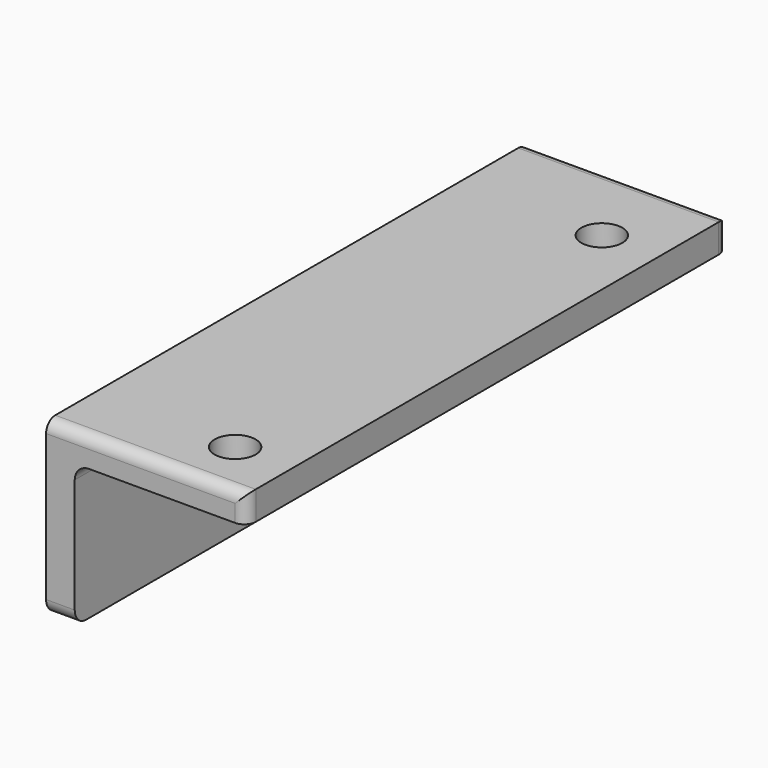
from build123d import *

# Parameters (mm, degrees)
F1_DEPTH = 133.35
F2_R     = 4.5466
F3_DEPTH = 25.4
F4_R     = 4.5466
F5_DEPTH = 25.4
F6_R     = 2.54
F7_R     = 3.175


with BuildPart() as f1:
    # F0 (on Front) → F1 (new body)
    with BuildSketch(Plane.XZ):
        Polygon((-29.6893073604, 12.910717619), (-29.6893073604, -25.189282381), (-23.3393073604, -25.189282381), (-23.3393073604, 6.560717619), (14.7606926396, 6.560717619), (14.7606926396, 12.910717619), align=None)
    extrude(amount=F1_DEPTH)

    # F2 (on face) → F3 (cut)
    with BuildSketch(Plane(origin=(-29.6893073604, 0, 0), x_dir=(0, -1, 0), z_dir=(-1, 0, 0))):
        with Locations((25.4, -14.076782381)):
            Circle(F2_R)
        with Locations((88.9, -14.076782381)):
            Circle(F2_R)
    extrude(amount=-F3_DEPTH, mode=Mode.SUBTRACT)

    # F4 (on face) → F5 (cut)
    with BuildSketch(Plane.XY.offset(12.910717619)):
        with Locations((2.0606926396, -120.65)):
            Circle(F4_R)
        with Locations((2.0606926396, -19.05)):
            Circle(F4_R)
    extrude(amount=-F5_DEPTH, mode=Mode.SUBTRACT)

    # F6
    f6_edges = [f1.edges().sort_by_distance(p)[0] for p in [
        (14.760693, -133.35, 9.735718),
        (-7.464307, -133.35, 12.910718),
        (-7.464307, 0, 12.910718),
        (14.760693, 0, 9.735718),
    ]]
    fillet(f6_edges, radius=F6_R)

    # F7
    f7_edges = [f1.edges().sort_by_distance(p)[0] for p in [
        (-26.514307, -133.35, -25.189282),
        (-26.514307, 0, -25.189282),
        (-23.339307, -66.675, 6.560718),
    ]]
    fillet(f7_edges, radius=F7_R)


solid = f1.part
